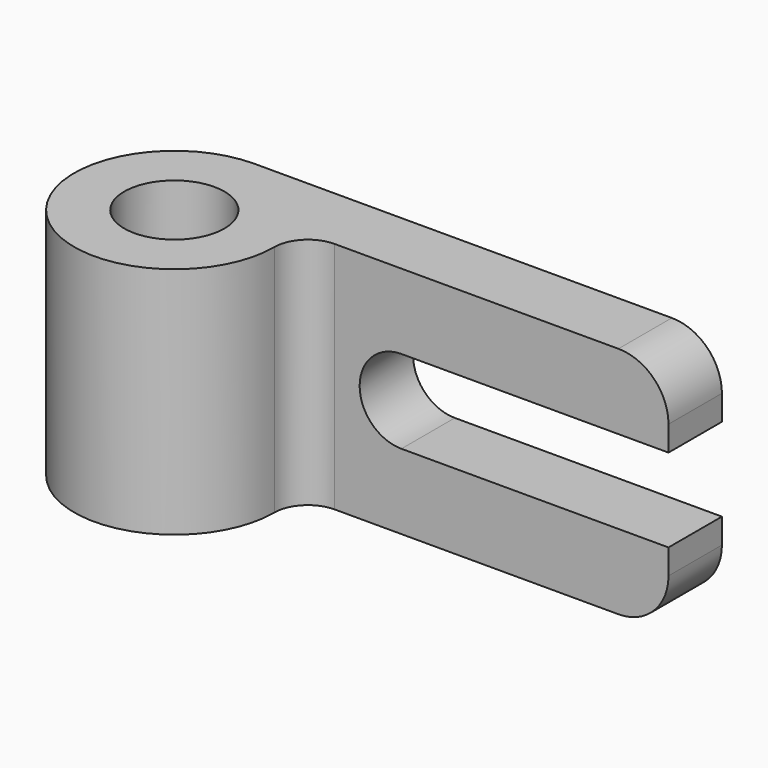
from build123d import *

# Parameters (mm, degrees)
F0_R     = 9.525
F1_DEPTH = 44.45
F3_DEPTH = 19.051
F4_R     = 9.525
F5_R     = 6.35


# Not quite as in the source:
# - a length typed as a fraction of an inch, garbled in the dataset ("3 / 203.2 mm" for 3/8 in), is restored


with BuildPart() as f1:
    # F0 (on Top) → F1 (new body)
    with BuildSketch(Plane.XY):
        with BuildLine():
            Line((88.9, 19.05), (0, 19.05))
            ThreePointArc((0, 19.05), (-10.9985226281, -15.5542598667), (17.9605122421, 6.35))
            Line((17.9605122421, 6.35), (88.9, 6.35))
            Line((88.9, 6.35), (88.9, 19.05))
        make_face()
        Circle(F0_R, mode=Mode.SUBTRACT)
    extrude(amount=F1_DEPTH)

    # F2 (on Front) → F3 (cut, through all)
    with BuildSketch(Plane.XZ):
        with BuildLine():
            Line((88.9, 14.2875), (88.9, 30.1625))
            Line((88.9, 30.1625), (38.1, 30.1625))
            ThreePointArc((38.1, 30.1625), (30.1625, 22.225), (38.1, 14.2875))
            Line((38.1, 14.2875), (88.9, 14.2875))
        make_face()
    extrude(amount=-F3_DEPTH, mode=Mode.SUBTRACT)

    # F4
    f4_edges = [f1.edges().sort_by_distance(p)[0] for p in [
        (88.9, 12.7, 44.45),
        (88.9, 12.7, 0),
    ]]
    fillet(f4_edges, radius=F4_R)

    # F5
    f5_edges = [f1.edges().sort_by_distance(p)[0] for p in [
        (17.960512, 6.35, 22.225),
    ]]
    fillet(f5_edges, radius=F5_R)


solid = f1.part
